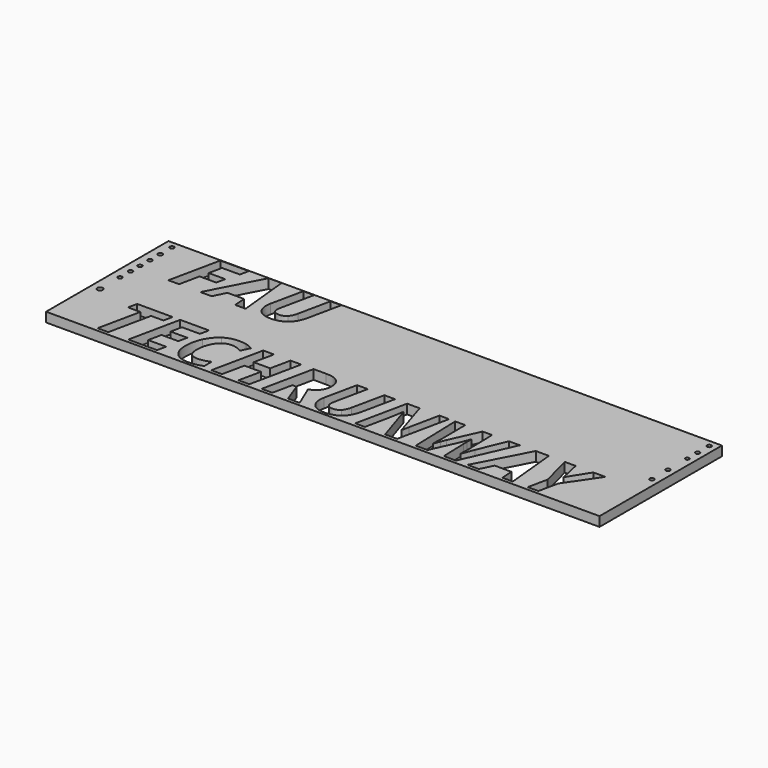
from build123d import *

# Parameters (mm, degrees)
F0_W     = 103.5013049841
F0_H     = 28.6082277307
F0_R     = 0.5104813739
F0_R_2   = 0.3994544341
F0_R_3   = 0.4006799492
F0_R_4   = 0.4083576228
F0_R_5   = 0.4059938545
F0_R_6   = 0.408233285
F0_R_7   = 0.4113471237
F0_R_8   = 0.4080996046
F0_R_9   = 0.4042135091
F0_R_10  = 0.3513599071
F0_R_11  = 0.3942156176
F0_R_12  = 0.4049216731
F1_DEPTH = 1.778


with BuildPart() as f1:
    # F0 (on Top) → F1 (new body)
    with BuildSketch(Plane.XY):
        with Locations((-0.5814656615, 11.0478929128)):
            Rectangle(F0_W, F0_H)
        Polygon((-39.5282860249, 5.2799193943), (-41.1972814572, -2.6299418294), (-43.2004963778, -2.6299418294), (-41.5315009455, 5.2799193943), (-43.8437112421, 5.2799193943), (-43.4821656321, 6.9741389389), (-36.8482240902, 6.9741389389), (-37.2097697002, 5.2799193943), align=None, mode=Mode.SUBTRACT)
        Polygon((-31.7361373254, -0.9483343409), (-32.0913769073, -2.6299418294), (-37.4578068048, -2.6299418294), (-35.4293677719, 6.9741389389), (-30.054529837, 6.9741389389), (-30.4097694189, 5.3051435067), (-33.7729843958, 5.3051435067), (-34.2144063615, 3.1968281181), (-31.0803104049, 3.1968281181), (-31.4418560149, 1.5278326858), (-34.5738499621, 1.5278326858), (-35.0993523023, -0.9483343409), align=None, mode=Mode.SUBTRACT)
        with BuildLine():
            add(Edge.make_bspline(
                [(-23.6696764043, 5.3051435067), (-24.1226594215, 5.4291620589), (-24.5703874153, 5.4291620589)],
                knots=[0, 0, 0, 1, 1, 1], degree=2))
            add(Edge.make_bspline(
                [(-24.5703874153, 5.4291620589), (-25.4364152719, 5.4291620589), (-26.1300783608, 4.8973536907)],
                knots=[0, 0, 0, 1, 1, 1], degree=2))
            add(Edge.make_bspline(
                [(-26.1300783608, 4.8973536907), (-26.8237414498, 4.3655453225), (-27.2441433219, 3.3313567171)],
                knots=[0, 0, 0, 1, 1, 1], degree=2))
            add(Edge.make_bspline(
                [(-27.2441433219, 3.3313567171), (-27.664545194, 2.2971681117), (-27.664545194, 1.1074308137)],
                knots=[0, 0, 0, 1, 1, 1], degree=2))
            add(Edge.make_bspline(
                [(-27.664545194, 1.1074308137), (-27.664545194, 0.0101819275), (-27.2147151909, -0.5216264407)],
                knots=[0, 0, 0, 1, 1, 1], degree=2))
            add(Edge.make_bspline(
                [(-27.2147151909, -0.5216264407), (-26.7648851877, -1.053434809), (-25.7790427976, -1.053434809)],
                knots=[0, 0, 0, 1, 1, 1], degree=2))
            add(Edge.make_bspline(
                [(-25.7790427976, -1.053434809), (-24.8205265292, -1.053434809), (-23.5593209129, -0.5468505531)],
                knots=[0, 0, 0, 1, 1, 1], degree=2))
            Line((-23.5593209129, -0.5468505531), (-23.5593209129, -2.2557841632))
            add(Edge.make_bspline(
                [(-23.5593209129, -2.2557841632), (-24.8646687258, -2.7623684191), (-26.1868326136, -2.7623684191)],
                knots=[0, 0, 0, 1, 1, 1], degree=2))
            add(Edge.make_bspline(
                [(-26.1868326136, -2.7623684191), (-27.8537260365, -2.7623684191), (-28.7807121645, -1.779679043)],
                knots=[0, 0, 0, 1, 1, 1], degree=2))
            add(Edge.make_bspline(
                [(-28.7807121645, -1.779679043), (-29.7076982925, -0.796989667), (-29.7076982925, 1.0023303457)],
                knots=[0, 0, 0, 1, 1, 1], degree=2))
            add(Edge.make_bspline(
                [(-29.7076982925, 1.0023303457), (-29.7076982925, 2.7238760119), (-29.0245452503, 4.1721604613)],
                knots=[0, 0, 0, 1, 1, 1], degree=2))
            add(Edge.make_bspline(
                [(-29.0245452503, 4.1721604613), (-28.3413922081, 5.6204449108), (-27.197899116, 6.3729642618)],
                knots=[0, 0, 0, 1, 1, 1], degree=2))
            add(Edge.make_bspline(
                [(-27.197899116, 6.3729642618), (-26.0544060239, 7.1254836129), (-24.5703874153, 7.1254836129)],
                knots=[0, 0, 0, 1, 1, 1], degree=2))
            add(Edge.make_bspline(
                [(-24.5703874153, 7.1254836129), (-23.7485017554, 7.1254836129), (-23.1115929191, 6.977291953)],
                knots=[0, 0, 0, 1, 1, 1], degree=2))
            add(Edge.make_bspline(
                [(-23.1115929191, 6.977291953), (-22.4746840829, 6.8291002931), (-21.7452868348, 6.4360245426)],
                knots=[0, 0, 0, 1, 1, 1], degree=2))
            Line((-21.7452868348, 6.4360245426), (-22.5209282888, 4.7922532227))
            add(Edge.make_bspline(
                [(-22.5209282888, 4.7922532227), (-23.2166933871, 5.1811249544), (-23.6696764043, 5.3051435067)],
                knots=[0, 0, 0, 1, 1, 1], degree=2))
        make_face(mode=Mode.SUBTRACT)
        Polygon((-12.797032987, 6.9741389389), (-14.8275740292, -2.6299418294), (-16.8370949779, -2.6299418294), (-15.9584550652, 1.5152206296), (-19.0505108346, 1.5152206296), (-19.9312527566, -2.6299418294), (-21.9344676772, -2.6299418294), (-19.9060286443, 6.9741389389), (-17.8944056863, 6.9741389389), (-18.6910672339, 3.2094401742), (-15.5969094552, 3.2094401742), (-14.8023499169, 6.9741389389), align=None, mode=Mode.SUBTRACT)
        with BuildLine():
            Line((-8.9482538478, 1.0548805797), (-9.7302013299, 1.0548805797))
            Line((-9.7302013299, 1.0548805797), (-10.512148812, -2.6299418294))
            Line((-10.512148812, -2.6299418294), (-12.5153637326, -2.6299418294))
            Line((-12.5153637326, -2.6299418294), (-10.4869246997, 6.9741389389))
            Line((-10.4869246997, 6.9741389389), (-8.1284701972, 6.9741389389))
            add(Edge.make_bspline(
                [(-8.1284701972, 6.9741389389), (-6.570881261, 6.9741389389), (-5.7889337789, 6.3035979529)],
                knots=[0, 0, 0, 1, 1, 1], degree=2))
            add(Edge.make_bspline(
                [(-5.7889337789, 6.3035979529), (-5.0069862968, 5.6330569669), (-5.0069862968, 4.3403212102)],
                knots=[0, 0, 0, 1, 1, 1], degree=2))
            add(Edge.make_bspline(
                [(-5.0069862968, 4.3403212102), (-5.0069862968, 3.3019285861), (-5.5524577259, 2.5567662678)],
                knots=[0, 0, 0, 1, 1, 1], degree=2))
            add(Edge.make_bspline(
                [(-5.5524577259, 2.5567662678), (-6.0979291549, 1.8116039495), (-7.1237097229, 1.4500583394)],
                knots=[0, 0, 0, 1, 1, 1], degree=2))
            Line((-7.1237097229, 1.4500583394), (-5.4084700847, -2.6299418294))
            Line((-5.4084700847, -2.6299418294), (-7.5903558009, -2.6299418294))
            Line((-7.5903558009, -2.6299418294), (-8.9482538478, 1.0548805797))
        make_face(mode=Mode.SUBTRACT)
        with Locations((-50.6688654423, 7.3013389483)):
            Circle(F0_R, mode=Mode.SUBTRACT)
        with BuildLine():
            Line((2.7368161874, 6.9741389389), (4.7463371361, 6.9741389389))
            Line((4.7463371361, 6.9741389389), (3.4262752577, 0.7605992692))
            add(Edge.make_bspline(
                [(3.4262752577, 0.7605992692), (3.0521175915, -0.9882725188), (1.9948068832, -1.8753204689)],
                knots=[0, 0, 0, 1, 1, 1], degree=2))
            add(Edge.make_bspline(
                [(1.9948068832, -1.8753204689), (0.9374961748, -2.7623684191), (-0.7567233698, -2.7623684191)],
                knots=[0, 0, 0, 1, 1, 1], degree=2))
            add(Edge.make_bspline(
                [(-0.7567233698, -2.7623684191), (-2.1503555758, -2.7623684191), (-2.9480681282, -2.0161550961)],
                knots=[0, 0, 0, 1, 1, 1], degree=2))
            add(Edge.make_bspline(
                [(-2.9480681282, -2.0161550961), (-3.7457806805, -1.2699417731), (-3.7457806805, 0.0038758994)],
                knots=[0, 0, 0, 1, 1, 1], degree=2))
            add(Edge.make_bspline(
                [(-3.7457806805, 0.0038758994), (-3.7457806805, 0.4768280055), (-3.6469862405, 0.9098419338)],
                knots=[0, 0, 0, 1, 1, 1], degree=2))
            Line((-3.6469862405, 0.9098419338), (-2.3605565119, 6.9741389389))
            Line((-2.3605565119, 6.9741389389), (-0.3573415913, 6.9741389389))
            Line((-0.3573415913, 6.9741389389), (-1.6311592638, 0.9371680555))
            add(Edge.make_bspline(
                [(-1.6311592638, 0.9371680555), (-1.7425657599, 0.4516038932), (-1.7425657599, 0.1152823955)],
                knots=[0, 0, 0, 1, 1, 1], degree=2))
            add(Edge.make_bspline(
                [(-1.7425657599, 0.1152823955), (-1.7425657599, -1.053434809), (-0.5023802372, -1.053434809)],
                knots=[0, 0, 0, 1, 1, 1], degree=2))
            add(Edge.make_bspline(
                [(-0.5023802372, -1.053434809), (0.3068933666, -1.053434809), (0.7798454728, -0.5510545718)],
                knots=[0, 0, 0, 1, 1, 1], degree=2))
            add(Edge.make_bspline(
                [(0.7798454728, -0.5510545718), (1.2527975789, -0.0486743346), (1.4629985149, 0.9497801116)],
                knots=[0, 0, 0, 1, 1, 1], degree=2))
            Line((1.4629985149, 0.9497801116), (2.7368161874, 6.9741389389))
        make_face(mode=Mode.SUBTRACT)
        with BuildLine():
            Line((14.8443901041, 6.9741389389), (12.8138490618, -2.6299418294))
            Line((12.8138490618, -2.6299418294), (10.5668010554, -2.6299418294))
            Line((10.5668010554, -2.6299418294), (8.2293666465, 4.6346025207))
            Line((8.2293666465, 4.6346025207), (8.1894284687, 4.6346025207))
            Line((8.1894284687, 4.6346025207), (8.162102347, 4.4244015846))
            add(Edge.make_bspline(
                [(8.162102347, 4.4244015846), (7.9519014109, 3.0055452662), (7.7290884187, 1.8893782958)],
                knots=[0, 0, 0, 1, 1, 1], degree=2))
            Line((7.7290884187, 1.8893782958), (6.7768781784, -2.6299418294))
            Line((6.7768781784, -2.6299418294), (4.9712521377, -2.6299418294))
            Line((4.9712521377, -2.6299418294), (6.9996911706, 6.9741389389))
            Line((6.9996911706, 6.9741389389), (9.345533617, 6.9741389389))
            Line((9.345533617, 6.9741389389), (11.5778675578, -0.1012245686))
            Line((11.5778675578, -0.1012245686), (11.6051936795, -0.1012245686))
            add(Edge.make_bspline(
                [(11.6051936795, -0.1012245686), (11.6829680259, 0.3990536592), (11.8605878168, 1.3249887825)],
                knots=[0, 0, 0, 1, 1, 1], degree=2))
            add(Edge.make_bspline(
                [(11.8605878168, 1.3249887825), (12.0382076078, 2.2509239058), (13.0429680821, 6.9741389389)],
                knots=[0, 0, 0, 1, 1, 1], degree=2))
            Line((13.0429680821, 6.9741389389), (14.8443901041, 6.9741389389))
        make_face(mode=Mode.SUBTRACT)
        with BuildLine():
            Line((21.4110673464, 4.0565499465), (21.3858432341, 4.0565499465))
            add(Edge.make_bspline(
                [(21.3858432341, 4.0565499465), (21.0831538862, 3.0980336781), (20.6291198643, 2.0932732038)],
                knots=[0, 0, 0, 1, 1, 1], degree=2))
            Line((20.6291198643, 2.0932732038), (18.5018863915, -2.6299418294))
            Line((18.5018863915, -2.6299418294), (16.2821645067, -2.6299418294))
            Line((16.2821645067, -2.6299418294), (15.9857811869, 6.9741389389))
            Line((15.9857811869, 6.9741389389), (17.8712835833, 6.9741389389))
            Line((17.8712835833, 6.9741389389), (17.9112217611, 1.7317275938))
            add(Edge.make_bspline(
                [(17.9112217611, 1.7317275938), (17.9112217611, 1.3912020774), (17.8849466441, 0.5955915344)],
                knots=[0, 0, 0, 1, 1, 1], degree=2))
            add(Edge.make_bspline(
                [(17.8849466441, 0.5955915344), (17.8586715271, -0.2000190086), (17.8187333493, -0.5468505531)],
                knots=[0, 0, 0, 1, 1, 1], degree=2))
            Line((17.8187333493, -0.5468505531), (17.8586715271, -0.5468505531))
            add(Edge.make_bspline(
                [(17.8586715271, -0.5468505531), (18.0016081636, -0.126448681), (18.2979914835, 0.6386827263)],
                knots=[0, 0, 0, 1, 1, 1], degree=2))
            add(Edge.make_bspline(
                [(18.2979914835, 0.6386827263), (18.5943748033, 1.4038141335), (18.6931692433, 1.592994976)],
                knots=[0, 0, 0, 1, 1, 1], degree=2))
            Line((18.6931692433, 1.592994976), (21.116786036, 6.9741389389))
            Line((21.116786036, 6.9741389389), (22.8887799269, 6.9741389389))
            Line((22.8887799269, 6.9741389389), (23.0275125447, 1.2398574034))
            add(Edge.make_bspline(
                [(23.0275125447, 1.2398574034), (23.0275125447, 0.2792391256), (22.9686562826, -0.5468505531)],
                knots=[0, 0, 0, 1, 1, 1], degree=2))
            Line((22.9686562826, -0.5468505531), (23.0085944604, -0.5468505531))
            add(Edge.make_bspline(
                [(23.0085944604, -0.5468505531), (23.2902637148, 0.3002592192), (23.8683162889, 1.7443396499)],
                knots=[0, 0, 0, 1, 1, 1], degree=2))
            Line((23.8683162889, 1.7443396499), (26.0354879396, 6.9741389389))
            Line((26.0354879396, 6.9741389389), (28.0660289819, 6.9741389389))
            Line((28.0660289819, 6.9741389389), (23.8157660549, -2.6299418294))
            Line((23.8157660549, -2.6299418294), (21.5434939361, -2.6299418294))
            Line((21.5434939361, -2.6299418294), (21.3984552903, 2.1058852599))
            Line((21.3984552903, 2.1058852599), (21.3858432341, 3.0202593318))
            add(Edge.make_bspline(
                [(21.3858432341, 3.0202593318), (21.3858432341, 3.5983119059), (21.4110673464, 4.0565499465)],
                knots=[0, 0, 0, 1, 1, 1], degree=2))
        make_face(mode=Mode.SUBTRACT)
        Polygon((32.4928606952, -2.6299418294), (32.3352099931, -0.3429556451), (29.2284401583, -0.3429556451), (28.0996611317, -2.6299418294), (25.9976517711, -2.6299418294), (31.0277601709, 7.0140771168), (33.4787030853, 7.0140771168), (34.4435253818, -2.6299418294), align=None, mode=Mode.SUBTRACT)
        Polygon((38.5235255506, 6.9741389389), (39.3706353229, 3.0854216219), (41.8278842653, 6.9741389389), (44.0749322718, 6.9741389389), (40.0159521966, 1.0422685235), (39.2340047144, -2.6299418294), (37.24340185, -2.6299418294), (38.0253493321, 1.0422685235), (36.474066424, 6.9741389389), align=None, mode=Mode.SUBTRACT)
        with Locations((49.8356483877, 10.640562512)):
            Circle(F0_R_2, mode=Mode.SUBTRACT)
        with Locations((-50.6688654423, 11.9424648583)):
            Circle(F0_R_3, mode=Mode.SUBTRACT)
        with Locations((-50.6688654423, 14.4119979814)):
            Circle(F0_R_4, mode=Mode.SUBTRACT)
        with Locations((-50.6688654423, 16.6217070073)):
            Circle(F0_R_5, mode=Mode.SUBTRACT)
        with Locations((-50.6688654423, 18.9477130771)):
            Circle(F0_R_6, mode=Mode.SUBTRACT)
        with Locations((-50.6688654423, 21.3609486818)):
            Circle(F0_R_7, mode=Mode.SUBTRACT)
        Polygon((-41.8005581437, 19.4621765499), (-42.5951176819, 15.6659476448), (-44.5983326025, 15.6659476448), (-42.5698935696, 25.2700284131), (-37.2223817564, 25.2700284131), (-37.5776213383, 23.6010329808), (-40.9135101935, 23.6010329808), (-41.4327065056, 21.1248659541), (-38.3259366707, 21.1248659541), (-38.6937883088, 19.4621765499), align=None, mode=Mode.SUBTRACT)
        Polygon((-32.118703029, 15.6659476448), (-32.2763537311, 17.952933829), (-35.3831235659, 17.952933829), (-36.5119025925, 15.6659476448), (-38.6139119531, 15.6659476448), (-33.5838035533, 25.3099665909), (-31.1328606389, 25.3099665909), (-30.1680383424, 15.6659476448), align=None, mode=Mode.SUBTRACT)
        with Locations((-50.6688654423, 24.0940079093)):
            Circle(F0_R_8, mode=Mode.SUBTRACT)
        with BuildLine():
            Line((-21.9491817427, 25.2700284131), (-19.9396607941, 25.2700284131))
            Line((-19.9396607941, 25.2700284131), (-21.2597226725, 19.0564887433))
            add(Edge.make_bspline(
                [(-21.2597226725, 19.0564887433), (-21.6338803387, 17.3076169553), (-22.691191047, 16.4205690052)],
                knots=[0, 0, 0, 1, 1, 1], degree=2))
            add(Edge.make_bspline(
                [(-22.691191047, 16.4205690052), (-23.7485017554, 15.533521055), (-25.4427212999, 15.533521055)],
                knots=[0, 0, 0, 1, 1, 1], degree=2))
            add(Edge.make_bspline(
                [(-25.4427212999, 15.533521055), (-26.836353506, 15.533521055), (-27.6340660583, 16.279734378)],
                knots=[0, 0, 0, 1, 1, 1], degree=2))
            add(Edge.make_bspline(
                [(-27.6340660583, 16.279734378), (-28.4317786106, 17.025947701), (-28.4317786106, 18.2997653735)],
                knots=[0, 0, 0, 1, 1, 1], degree=2))
            add(Edge.make_bspline(
                [(-28.4317786106, 18.2997653735), (-28.4317786106, 18.7727174796), (-28.3329841707, 19.2057314079)],
                knots=[0, 0, 0, 1, 1, 1], degree=2))
            Line((-28.3329841707, 19.2057314079), (-27.046554442, 25.2700284131))
            Line((-27.046554442, 25.2700284131), (-25.0433395214, 25.2700284131))
            Line((-25.0433395214, 25.2700284131), (-26.3171571939, 19.2330575296))
            add(Edge.make_bspline(
                [(-26.3171571939, 19.2330575296), (-26.42856369, 18.7474933673), (-26.42856369, 18.4111718696)],
                knots=[0, 0, 0, 1, 1, 1], degree=2))
            add(Edge.make_bspline(
                [(-26.42856369, 18.4111718696), (-26.42856369, 17.2424546652), (-25.1883781673, 17.2424546652)],
                knots=[0, 0, 0, 1, 1, 1], degree=2))
            add(Edge.make_bspline(
                [(-25.1883781673, 17.2424546652), (-24.3791045635, 17.2424546652), (-23.9061524574, 17.7448349023)],
                knots=[0, 0, 0, 1, 1, 1], degree=2))
            add(Edge.make_bspline(
                [(-23.9061524574, 17.7448349023), (-23.4332003513, 18.2472151395), (-23.2229994152, 19.2456695858)],
                knots=[0, 0, 0, 1, 1, 1], degree=2))
            Line((-23.2229994152, 19.2456695858), (-21.9491817427, 25.2700284131))
        make_face(mode=Mode.SUBTRACT)
        with Locations((49.8356483877, 14.4119979814)):
            Circle(F0_R_9, mode=Mode.SUBTRACT)
        with Locations((49.8356483877, 18.9477130771)):
            Circle(F0_R_10, mode=Mode.SUBTRACT)
        with Locations((49.8356483877, 21.3609486818)):
            Circle(F0_R_11, mode=Mode.SUBTRACT)
        with Locations((49.8356483877, 24.0940079093)):
            Circle(F0_R_12, mode=Mode.SUBTRACT)
    extrude(amount=-F1_DEPTH)


solid = f1.part
